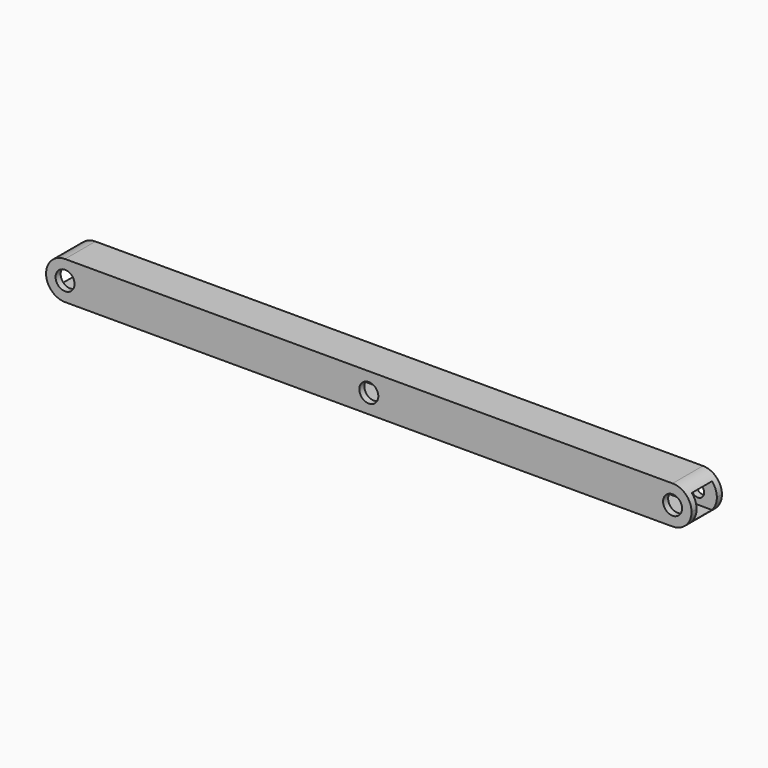
from build123d import *

# Parameters (mm, degrees)
F0_W        = 19.05
F0_H        = 19.05
F0_W_2      = 12.7
F0_H_2      = 12.7
F1_DEPTH    = 323.85
F3_T1_DEPTH = 66.675
F4_T1_DEPTH = 66.675
F2_R        = 3.175
F5_DEPTH    = 19.051
F2_R_2      = 4.7625
F6_DEPTH    = 3.175


# Not quite as in the source:
# - a fillet or chamfer that OpenCascade refuses, or shapes differently, is made with other operations: its cross-section is extruded or revolved along the edge and cut away or added


with BuildPart() as f1:
    # F0 (on Right) → F1 (new body)
    with BuildSketch(Plane.YZ):
        Rectangle(F0_W, F0_H)
        Rectangle(F0_W_2, F0_H_2, mode=Mode.SUBTRACT)
    extrude(amount=F1_DEPTH)

    # F3: fillet of radius 9.525 on 2 edges, made by hand

    # F3_s2 → F3_t1 (cut)
    with BuildSketch(Plane.XZ.offset(-33.3375)):
        with BuildLine():
            ThreePointArc((9.525, 9.525), (2.7898079092, 6.7351920908), (0, 0))
            Line((0, 0), (0, 9.525))
            Line((0, 9.525), (9.525, 9.525))
        make_face()
        with BuildLine():
            ThreePointArc((9.525, -9.525), (2.7898079092, -6.7351920908), (0, 0))
            Line((0, 0), (0, -9.525))
            Line((0, -9.525), (9.525, -9.525))
        make_face()
    extrude(amount=F3_T1_DEPTH, mode=Mode.SUBTRACT)

    # F4: fillet of radius 9.525 on 2 edges, made by hand

    # F4_s2 → F4_t1 (cut)
    with BuildSketch(Plane.XZ.offset(-33.3375)):
        with BuildLine():
            ThreePointArc((314.325, 9.525), (321.0601920908, 6.7351920908), (323.85, 0))
            Line((323.85, 0), (323.85, 9.525))
            Line((323.85, 9.525), (314.325, 9.525))
        make_face()
        with BuildLine():
            ThreePointArc((323.85, 0), (321.0601920908, -6.7351920908), (314.325, -9.525))
            Line((314.325, -9.525), (323.85, -9.525))
            Line((323.85, -9.525), (323.85, 0))
        make_face()
    extrude(amount=F4_T1_DEPTH, mode=Mode.SUBTRACT)

    # F2 (on face) → F5 (cut, through all)
    with BuildSketch(Plane.XZ.offset(9.525)):
        with Locations((314.325, 0)):
            Circle(F2_R)
        with Locations((161.925, 0)):
            Circle(F2_R)
        with Locations((9.525, 0)):
            Circle(F2_R)
    extrude(amount=-F5_DEPTH, mode=Mode.SUBTRACT)

    # F2 (on face) → F6 (cut, through all)
    with BuildSketch(Plane.XZ.offset(9.525)):
        with Locations((9.525, 0)):
            Circle(F2_R_2)
        with Locations((9.525, 0)):
            Circle(F2_R, mode=Mode.SUBTRACT)
        with Locations((161.925, 0)):
            Circle(F2_R_2)
        with Locations((161.925, 0)):
            Circle(F2_R, mode=Mode.SUBTRACT)
        with Locations((314.325, 0)):
            Circle(F2_R_2)
        with Locations((314.325, 0)):
            Circle(F2_R, mode=Mode.SUBTRACT)
    extrude(amount=-F6_DEPTH, mode=Mode.SUBTRACT)


solid = f1.part
